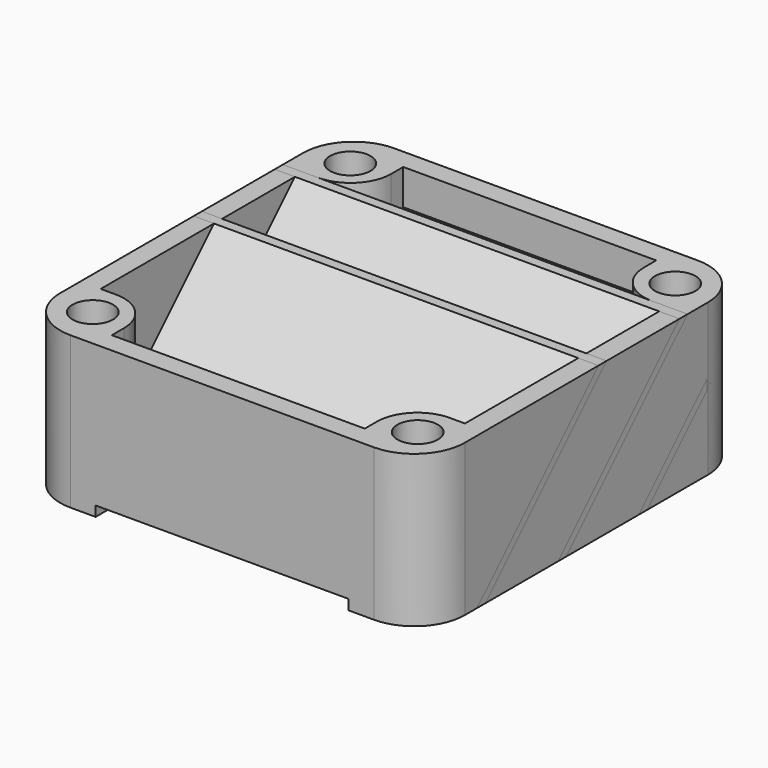
from build123d import *

# Parameters (mm, degrees)
F0_R        = 2
F0_W        = 25
F0_H        = 2
F0_W_2      = 2
F0_H_2      = 25
F1_DEPTH    = 15
F2_R        = 5
F3_R        = 4
F5_DEPTH    = 40
F6_T1_DEPTH = 26
F7_R        = 2
F8_DEPTH    = 25
F9_T1_DEPTH = 25


# Not quite as in the source:
# - a fillet or chamfer that OpenCascade refuses, or shapes differently, is made with other operations: its cross-section is extruded or revolved along the edge and cut away or added


with BuildPart() as f1:
    # F0 (on Top) → F1 (new body)
    with BuildSketch(Plane.XY):
        Polygon((-29.4209998254, 31.0463201136), (-21.9209998254, 31.0463201136), (-21.9209998254, 38.5463201136), (-23.9209998254, 38.5463201136), (-29.4209998254, 38.5463201136), (-29.4209998254, 33.0463201136), align=None)
        with Locations((-25.8659998254, 35.1404414833)):
            Circle(F0_R, mode=Mode.SUBTRACT)
        with Locations((-41.9209998254, 32.0463201136)):
            Rectangle(F0_W, F0_H)
        with Locations((-22.9209998254, 51.0463201136)):
            Rectangle(F0_W_2, F0_H_2)
        Polygon((-61.9209998254, 31.0463201136), (-54.4209998254, 31.0463201136), (-54.4209998254, 33.0463201136), (-54.4209998254, 38.5463201136), (-59.9209998254, 38.5463201136), (-61.9209998254, 38.5463201136), align=None)
        with Locations((-57.9759998254, 35.1404414833)):
            Circle(F0_R, mode=Mode.SUBTRACT)
        Polygon((-23.9209998254, 63.5463201136), (-21.9209998254, 63.5463201136), (-21.9209998254, 71.0463201136), (-29.4209998254, 71.0463201136), (-29.4209998254, 69.0463201136), (-29.4209998254, 63.5463201136), align=None)
        with Locations((-25.8659998254, 66.9521987438)):
            Circle(F0_R, mode=Mode.SUBTRACT)
        with Locations((-60.9209998254, 51.0463201136)):
            Rectangle(F0_W_2, F0_H_2)
        with Locations((-41.9209998254, 70.0463201136)):
            Rectangle(F0_W, F0_H)
        Polygon((-61.9209998254, 71.0463201136), (-61.9209998254, 63.5463201136), (-59.9209998254, 63.5463201136), (-54.4209998254, 63.5463201136), (-54.4209998254, 69.0463201136), (-54.4209998254, 71.0463201136), align=None)
        with Locations((-57.9759998254, 66.9521987438)):
            Circle(F0_R, mode=Mode.SUBTRACT)
    extrude(amount=F1_DEPTH)

    # F2
    f2_edges = [f1.edges().sort_by_distance(p)[0] for p in [
        (-61.921, 71.04632, 7.5),
        (-61.921, 31.04632, 7.5),
        (-21.921, 31.04632, 7.5),
        (-21.921, 71.04632, 7.5),
    ]]
    fillet(f2_edges, radius=F2_R)

    # F3
    f3_edges = [f1.edges().sort_by_distance(p)[0] for p in [
        (-54.421, 63.54632, 7.5),
        (-29.421, 63.54632, 7.5),
        (-29.421, 38.54632, 7.5),
        (-54.421, 38.54632, 7.5),
    ]]
    fillet(f3_edges, radius=F3_R)

    # F9: fillet of radius 5 on 1 edges, made by hand

    # F9_s2 → F9_t1 (cut)
    with BuildSketch(Plane.YZ.offset(-54.4209998254)):
        with BuildLine():
            ThreePointArc((28.0463201136, 0), (31.5818540195, 1.4644660941), (33.0463201136, 5))
            Line((33.0463201136, 5), (33.0463201136, 0))
            Line((33.0463201136, 0), (28.0463201136, 0))
        make_face()
    extrude(amount=F9_T1_DEPTH, mode=Mode.SUBTRACT)


with BuildPart() as f5:
    # F4 (on face) → F5 (new body)
    with BuildSketch(Plane(origin=(-61.9209998254, 0, 0), x_dir=(0, -1, 0), z_dir=(-1, 0, 0))):
        Polygon((-66.0463201136, 8.5), (-66.0463201136, 7.5), (-58.5463201136, 0), (-57.5463201136, 0), align=None)
        Polygon((-70.9395914093, 12.3932712957), (-66.0463201136, 7.5), (-66.0463201136, 8.5), (-70.9395914093, 13.3932712957), align=None)
    extrude(amount=-F5_DEPTH)

    # F6: fillet of radius 5 on 2 edges, made by hand

    # F6_s2 → F6_t1 (cut)
    with BuildSketch(Plane.XY.offset(-0.1067287043)):
        with BuildLine():
            ThreePointArc((-56.9209998254, 70.9395914093), (-60.4565337313, 69.4751253152), (-61.9209998254, 65.9395914093))
            Line((-61.9209998254, 65.9395914093), (-61.9209998254, 70.9395914093))
            Line((-61.9209998254, 70.9395914093), (-56.9209998254, 70.9395914093))
        make_face()
        with BuildLine():
            ThreePointArc((-26.9209998254, 70.9395914093), (-23.3854659194, 69.4751253152), (-21.9209998254, 65.9395914093))
            Line((-21.9209998254, 65.9395914093), (-21.9209998254, 70.9395914093))
            Line((-21.9209998254, 70.9395914093), (-26.9209998254, 70.9395914093))
        make_face()
    extrude(amount=F6_T1_DEPTH, mode=Mode.SUBTRACT)

    # F7 (on face) → F8 (cut)
    with BuildSketch(Plane(origin=(0, 0, 0), x_dir=(1, 0, 0), z_dir=(0, 0, -1))):
        with Locations((-25.8659998254, -66.9521987438)):
            Circle(F7_R)
        with Locations((-57.9759998254, -66.9521987438)):
            Circle(F7_R)
    extrude(amount=-F8_DEPTH, mode=Mode.SUBTRACT)


with BuildPart() as f5b:
    # F4 (on face) → F5, piece 2 (new body)
    with BuildSketch(Plane(origin=(-61.9209998254, 0, 0), x_dir=(0, -1, 0), z_dir=(-1, 0, 0))):
        Polygon((-63.5463201136, 15), (-56.0463201136, 7.5), (-48.5463201136, 0), (-47.5463201136, 0), (-56.0463201136, 8.5), (-62.5463201136, 15), align=None)
    extrude(amount=-F5_DEPTH)


with BuildPart() as f5c:
    # F4 (on face) → F5, piece 3 (new body)
    with BuildSketch(Plane(origin=(-61.9209998254, 0, 0), x_dir=(0, -1, 0), z_dir=(-1, 0, 0))):
        Polygon((-53.5463201136, 15), (-46.0463201136, 7.5), (-38.5463201136, 0), (-37.5463201136, 0), (-46.0463201136, 8.5), (-52.5463201136, 15), align=None)
    extrude(amount=-F5_DEPTH)


solid = Compound([f1.part, f5.part, f5b.part, f5c.part])
